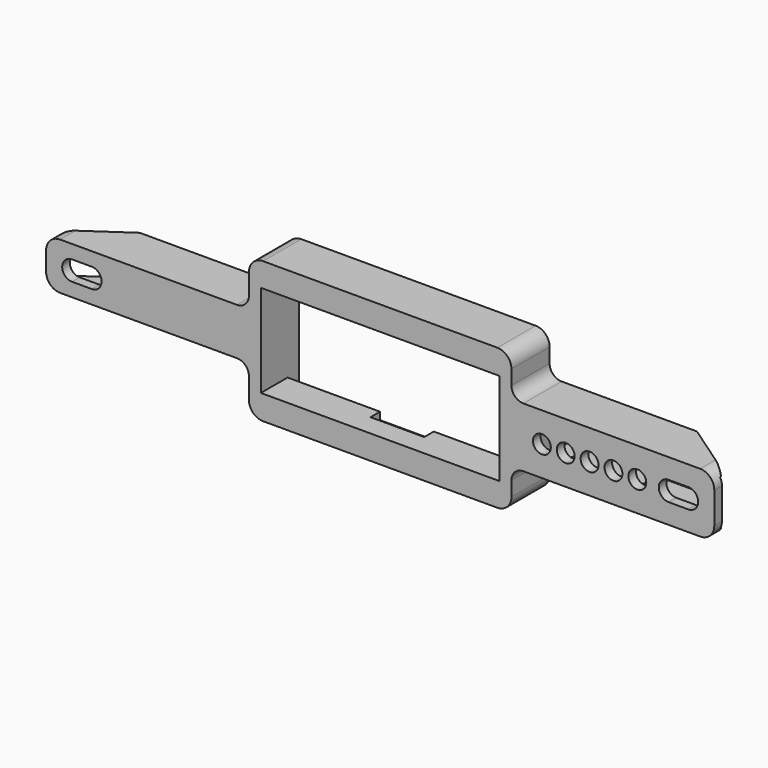
from build123d import *

# Parameters (mm, degrees)
F0_W         = 50.8
F0_H         = 19.7104
F0_W_2       = 43.18
F0_H_2       = 10
F0_H_3       = 12.7
F1_DEPTH     = 10.16
F2_W         = 50.8
F2_H         = 3.6068
F2_H_2       = 19.7104
F3_DEPTH     = 3.048
F4_W         = 45.72
F4_H         = 9.652
F4_W_2       = 2.54
F4_H_2       = 6.952
F4_W_3       = 12.7
F5_DEPTH     = 8.128
F8_DEPTH     = 25
F10_T1_DEPTH = 25.16
F10_T3_DEPTH = 17.032
F12_D        = 1.6
F12_DEPTH    = 5.842
F12_TIP      = 0.4806884952
F13_W        = 5.715
F13_H        = 3.6068
F14_DEPTH    = 2.54
F15_W        = 5.715
F15_H        = 3.6068
F16_DEPTH    = 2.54
F17_DEPTH    = 25.4
F18_R        = 2.54
F20_D        = 3.81
F21_W        = 6.35
F21_H        = 9.652
F22_W        = 6.35
F22_H        = 6.952
F23_DEPTH    = 8.128
F25_D        = 3.2639
F25_DEPTH    = 8.255
F25_TIP      = 0.9805744872


# Not quite as in the source:
# - a fillet or chamfer that OpenCascade refuses, or shapes differently, is made with other operations: its cross-section is extruded or revolved along the edge and cut away or added


with BuildPart() as f1:
    # F0 (on Front) → F1 (new body)
    with BuildSketch(Plane.XZ):
        Polygon((75.1493134361, 16.2306381539), (19.2693134361, 16.2306381539), (19.2693134361, 6.2332381539), (19.2693134361, -3.7667618461), (19.2693134361, -13.7667618461), (75.1493134361, -13.7667618461), (75.1493134361, -5.1180618461), (75.1493134361, 7.5819381539), align=None)
        with Locations((47.2093134361, 1.2319381539)):
            Rectangle(F0_W, F0_H, mode=Mode.SUBTRACT)
        with Locations((-2.3206865639, 1.2332381539)):
            Rectangle(F0_W_2, F0_H_2)
        with Locations((96.7393134361, 1.2319381539)):
            Rectangle(F0_W_2, F0_H_3)
    extrude(amount=-F1_DEPTH)

    # F2 (on face) → F3 (cut)
    with BuildSketch(Plane(origin=(0, 10.16, 0), x_dir=(-1, 0, 0), z_dir=(0, 1, 0))):
        with Locations((-47.2093134361, -10.4266618461)):
            Rectangle(F2_W, F2_H)
        with Locations((-47.2093134361, 1.2319381539)):
            Rectangle(F2_W, F2_H_2)
        with Locations((-47.2093134361, 12.8905381539)):
            Rectangle(F2_W, F2_H)
    extrude(amount=-F3_DEPTH, mode=Mode.SUBTRACT)

    # F4 (on face) → F5 (cut)
    with BuildSketch(Plane(origin=(0, 10.16, 0), x_dir=(-1, 0, 0), z_dir=(0, 1, 0))):
        with Locations((-95.4693134361, 1.2319381539)):
            Rectangle(F4_W, F4_H)
        with Locations((-71.3393134361, 1.2319381539)):
            Rectangle(F4_W_2, F4_H)
        with Locations((-23.0793134361, 1.2332381539)):
            Rectangle(F4_W_2, F4_H_2)
        with Locations((1.0506865639, 1.2332381539)):
            Rectangle(F4_W, F4_H_2)
        with Locations((30.2606865639, 1.2332381539)):
            Rectangle(F4_W_3, F4_H_2)
    extrude(amount=-F5_DEPTH, mode=Mode.SUBTRACT)

    # F7 (on face) + F6 (on face) → F8 (cut)
    with BuildSketch(Plane.XY.offset(6.2332381539)):
        Polygon((-23.9106865639, 10.16), (-23.9106865639, 2.032), (-12.0996865639, 10.16), align=None)
    with BuildSketch(Plane.XY.offset(7.5819381539)):
        Polygon((118.3293134361, 10.16), (106.5183134361, 10.16), (118.3293134361, 2.032), align=None)
    extrude(amount=-F8_DEPTH, mode=Mode.SUBTRACT)

    # F10: fillet of radius 3 on 8 edges, made by hand

    # F10_s2 → F10_t1 (cut)
    with BuildSketch(Plane.XZ.offset(-17.66)):
        with BuildLine():
            ThreePointArc((72.1493134361, -13.7667618461), (74.2706337797, -12.8880821896), (75.1493134361, -10.7667618461))
            Line((75.1493134361, -10.7667618461), (75.1493134361, -13.7667618461))
            Line((75.1493134361, -13.7667618461), (72.1493134361, -13.7667618461))
        make_face()
        with BuildLine():
            ThreePointArc((19.2693134361, -10.7667618461), (20.1479930925, -12.8880821896), (22.2693134361, -13.7667618461))
            Line((22.2693134361, -13.7667618461), (19.2693134361, -13.7667618461))
            Line((19.2693134361, -13.7667618461), (19.2693134361, -10.7667618461))
        make_face()
        with BuildLine():
            ThreePointArc((22.2693134361, 16.2306381539), (20.1479930925, 15.3519584975), (19.2693134361, 13.2306381539))
            Line((19.2693134361, 13.2306381539), (19.2693134361, 16.2306381539))
            Line((19.2693134361, 16.2306381539), (22.2693134361, 16.2306381539))
        make_face()
        with BuildLine():
            ThreePointArc((72.1493134361, 16.2306381539), (74.2706337797, 15.3519584975), (75.1493134361, 13.2306381539))
            Line((75.1493134361, 13.2306381539), (75.1493134361, 16.2306381539))
            Line((75.1493134361, 16.2306381539), (72.1493134361, 16.2306381539))
        make_face()
    extrude(amount=F10_T1_DEPTH, mode=Mode.SUBTRACT)

    # F10_s4 → F10_t3 (cut)
    with BuildSketch(Plane.XZ.offset(-9.532)):
        with BuildLine():
            ThreePointArc((-23.9106865639, -0.7667618461), (-23.0320069075, -2.8880821896), (-20.9106865639, -3.7667618461))
            Line((-20.9106865639, -3.7667618461), (-23.9106865639, -3.7667618461))
            Line((-23.9106865639, -3.7667618461), (-23.9106865639, -0.7667618461))
        make_face()
        with BuildLine():
            ThreePointArc((-20.9106865639, 6.2332381539), (-23.0320069075, 5.3545584975), (-23.9106865639, 3.2332381539))
            Line((-23.9106865639, 3.2332381539), (-23.9106865639, 6.2332381539))
            Line((-23.9106865639, 6.2332381539), (-20.9106865639, 6.2332381539))
        make_face()
        with BuildLine():
            ThreePointArc((115.3293134361, -5.1180618461), (117.4506337797, -4.2393821896), (118.3293134361, -2.1180618461))
            Line((118.3293134361, -2.1180618461), (118.3293134361, -5.1180618461))
            Line((118.3293134361, -5.1180618461), (115.3293134361, -5.1180618461))
        make_face()
        with BuildLine():
            ThreePointArc((115.3293134361, 7.5819381539), (117.4506337797, 6.7032584975), (118.3293134361, 4.5819381539))
            Line((118.3293134361, 4.5819381539), (118.3293134361, 7.5819381539))
            Line((118.3293134361, 7.5819381539), (115.3293134361, 7.5819381539))
        make_face()
    extrude(amount=F10_T3_DEPTH, mode=Mode.SUBTRACT)

    # F12
    with Locations(Plane(origin=(0, 7.112, 0), x_dir=(-1, 0, 0), z_dir=(0, 1, 0))):
        with Locations((-68.9771134361, 12.5857381539), (-25.4415134361, 12.5870381539), (-25.4415134361, -10.1205618461), (-68.9771134361, -10.1218618461)):
            Hole(F12_D / 2, depth=F12_DEPTH)
            with Locations((0, 0, -(F12_DEPTH + F12_TIP / 2))):  # 118° drill point
                Cone(0, F12_D / 2, F12_TIP, mode=Mode.SUBTRACT)

    # F13 (on face) → F14 (cut)
    with BuildSketch(Plane(origin=(0, 7.112, 0), x_dir=(-1, 0, 0), z_dir=(0, 1, 0))):
        with Locations((-50.0668134361, 12.8905381539)):
            Rectangle(F13_W, F13_H)
        with Locations((-44.3518134361, 12.8905381539)):
            Rectangle(F13_W, F13_H)
    extrude(amount=-F14_DEPTH, mode=Mode.SUBTRACT)

    # F15 (on face) → F16 (cut)
    with BuildSketch(Plane(origin=(0, 7.112, 0), x_dir=(-1, 0, 0), z_dir=(0, 1, 0))):
        with Locations((-50.0668134361, -10.4266618461)):
            Rectangle(F15_W, F15_H)
        with Locations((-44.3518134361, -10.4266618461)):
            Rectangle(F15_W, F15_H)
    extrude(amount=-F16_DEPTH, mode=Mode.SUBTRACT)

    # F9 (on face) → F17 (cut)
    with BuildSketch(Plane(origin=(0, 2.032, 0), x_dir=(-1, 0, 0), z_dir=(0, 1, 0))):
        with BuildLine():
            Line((-112.8048134361, -0.8584618461), (-108.6138134361, -0.8584618461))
            ThreePointArc((-108.6138134361, -0.8584618461), (-106.5183134361, 1.2370381539), (-108.6138134361, 3.3325381539))
            Line((-108.6138134361, 3.3325381539), (-112.8048134361, 3.3325381539))
            ThreePointArc((-112.8048134361, 3.3325381539), (-114.9003134361, 1.2370381539), (-112.8048134361, -0.8584618461))
        make_face()
        with BuildLine():
            Line((18.3861865639, 3.3325381428), (14.1951865639, 3.3325381428))
            ThreePointArc((14.1951865639, 3.3325381428), (12.0996865639, 1.2370381428), (14.1951865639, -0.8584618572))
            Line((14.1951865639, -0.8584618572), (18.3861865639, -0.8584618572))
            ThreePointArc((18.3861865639, -0.8584618572), (20.4816865639, 1.2370381428), (18.3861865639, 3.3325381428))
        make_face()
    extrude(amount=-F17_DEPTH, mode=Mode.SUBTRACT)

    # F18
    f18_edges = [f1.edges().sort_by_distance(p)[0] for p in [
        (75.149313, 5.08, 7.581938),
        (75.149313, 5.08, -5.118062),
        (19.269313, 5.08, 6.233238),
        (19.269313, 5.08, -3.766762),
    ]]
    fillet(f18_edges, radius=F18_R)

    # F20 (through all)
    with Locations(Plane(origin=(0, 2.032, 0), x_dir=(-1, 0, 0), z_dir=(0, 1, 0))):
        with Locations((-101.9463134361, 1.2319381539), (-91.7863134361, 1.2319381539), (-81.6263134361, 1.2319381539), (-86.7063134361, 1.2319381539), (-96.8663134361, 1.2319381539)):
            Hole(F20_D / 2)

    # F21 (on face) + F22 (on face) → F23 (join)
    with BuildSketch(Plane(origin=(0, 2.032, 0), x_dir=(-1, 0, 0), z_dir=(0, 1, 0))):
        with Locations((-75.7843134361, 1.2319381539)):
            Rectangle(F21_W, F21_H)
    with BuildSketch(Plane(origin=(0, 2.032, 0), x_dir=(-1, 0, 0), z_dir=(0, 1, 0))):
        with Locations((-18.6343134361, 1.2332381539)):
            Rectangle(F22_W, F22_H)
    extrude(amount=F23_DEPTH)

    # F25
    with Locations(Plane(origin=(0, 0, -5.1180618461), x_dir=(1, 0, 0), z_dir=(0, 0, -1))):
        with Locations((84.1663134361, -6.223), (99.4063134361, -6.223)):
            Hole(F25_D / 2, depth=F25_DEPTH)
            with Locations((0, 0, -(F25_DEPTH + F25_TIP / 2))):  # 118° drill point
                Cone(0, F25_D / 2, F25_TIP, mode=Mode.SUBTRACT)


solid = f1.part
